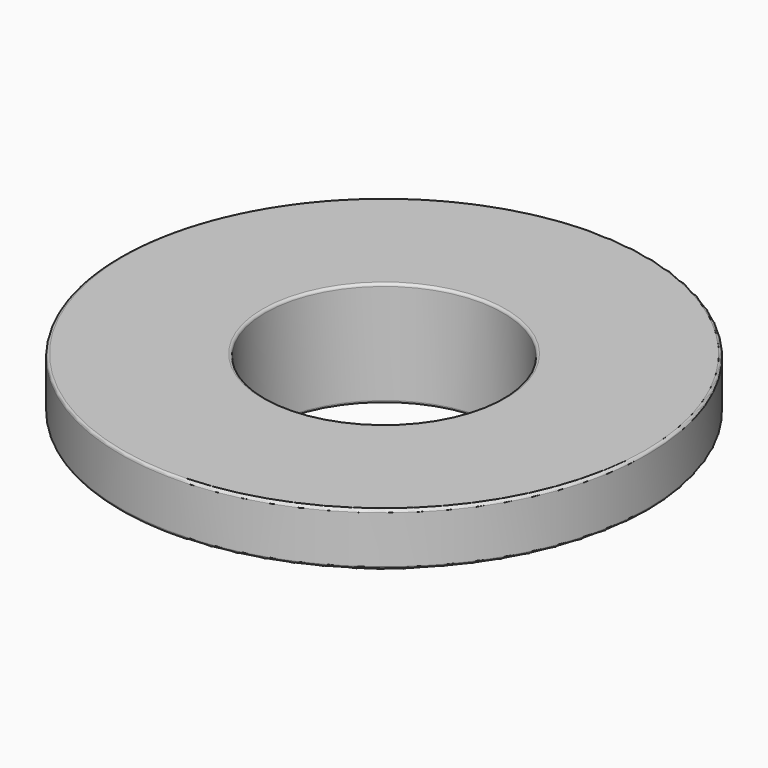
from build123d import *

# Parameters (mm, degrees)
F0_R     = 6.2
F1_DEPTH = 2
F2_R     = 10
F2_R_2   = 6.2
F3_DEPTH = 2
F5_D     = 9
F6_R     = 0.1


with BuildPart() as f1:
    # F0 (on Top) → F1 (new body)
    with BuildSketch(Plane.XY):
        Circle(F0_R)
    extrude(amount=F1_DEPTH)

    # F2 (on face) → F3 (join)
    with BuildSketch(Plane.XY.offset(2)):
        Circle(F2_R)
        Circle(F2_R_2, mode=Mode.SUBTRACT)
        Circle(F2_R_2)
    extrude(amount=F3_DEPTH)

    # F5 (through all)
    with Locations(Plane.XY.offset(4)):
        with Locations((0, 0)):
            Hole(F5_D / 2)

    # F6
    f6_edges = [f1.edges().sort_by_distance(p)[0] for p in [
        (-10, 0, 4),
        (-10, 0, 2),
        (-6.2, 0, 0),
        (-6.2, 0, 2),
        (-4.5, 0, 4),
        (-4.5, 0, 0),
    ]]
    fillet(f6_edges, radius=F6_R)


solid = f1.part
